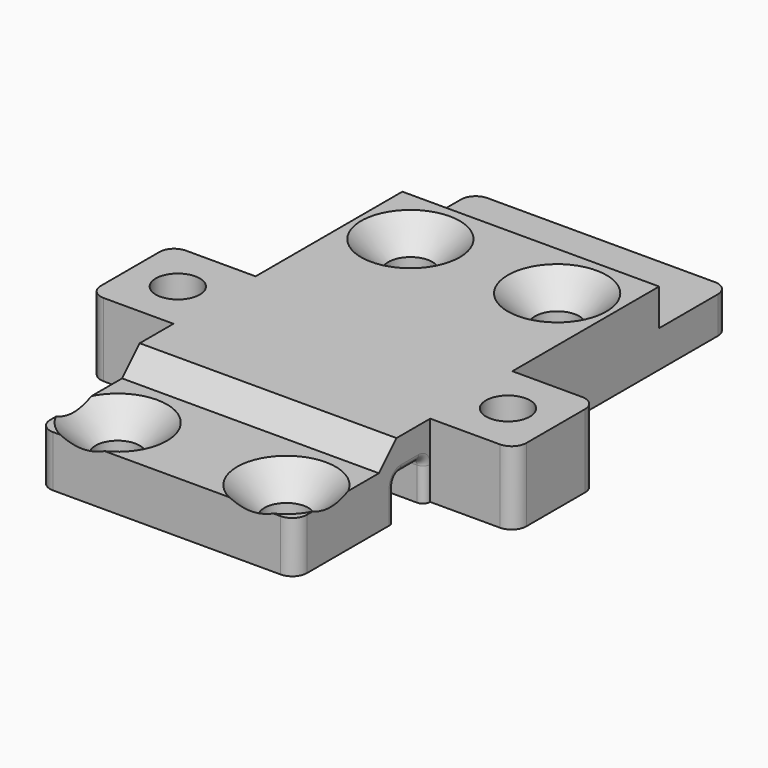
from build123d import *

# Parameters (mm, degrees)
F0_W            = 11.5
F0_H            = 14
F1_DEPTH        = 10
F2_W            = 5
F2_H            = 5.5
F2_H_2          = 4
F2_W_2          = 12
F2_H_3          = 5
F3_DEPTH        = 17.501
F7_D            = 5
F8_D            = 6
F9_D            = 6
F9_CSINK_D      = 13.44
F9_CSINK_ANGLE  = 90
F11_D           = 6
F11_CSINK_D     = 13.44
F11_CSINK_ANGLE = 90
F12_R           = 2
F13_R           = 0.99999


# Not quite as in the source:
# - a fillet or chamfer is up to 0.001 mm smaller than in the source, because OpenCascade refuses the exact size


with BuildPart() as f1:
    # F0 (on Top) → F1 (new body)
    with BuildSketch(Plane.XY):
        with Locations((23.25, 4.2037045646)):
            Rectangle(F0_W, F0_H)
        Polygon((17.5, 48.2037045646), (0, 48.2037045646), (0, -25.7962954354), (17.5, -25.7962954354), (17.5, -2.7962954354), (17.5, 11.2037045646), align=None)
    extrude(amount=F1_DEPTH)

    # F2 (on face) → F3 (cut, through all)
    with BuildSketch(Plane.YZ.offset(17.5)):
        Polygon((-25.7962954354, 10), (-25.7962954354, 7), (-11.5389361225, 7), (-8.5389361225, 10), align=None)
        with Locations((-6.2962954354, 2.75)):
            Rectangle(F2_W, F2_H)
        with Locations((13.7037045646, 2)):
            Rectangle(F2_W, F2_H_2)
        with Locations((42.2037045646, 7.5)):
            Rectangle(F2_W_2, F2_H_3)
    extrude(amount=-F3_DEPTH, mode=Mode.SUBTRACT)

    # F7 (through all)
    with Locations(Plane.XY.offset(5)):
        with Locations((10, 41.2037045646)):
            Hole(F7_D / 2)

    # F8 (through all)
    with Locations(Plane.XY.offset(10)):
        with Locations((22.5, 4.2037045646)):
            Hole(F8_D / 2)

    # F9 (through all)
    with Locations(Plane.XY.offset(7)):
        with Locations((11.5, -19.7962954354)):
            CounterSinkHole(F9_D / 2, F9_CSINK_D / 2, counter_sink_angle=F9_CSINK_ANGLE)

    # F11 (through all)
    with Locations(Plane.XY.offset(10)):
        with Locations((10, 28.2037045646)):
            CounterSinkHole(F11_D / 2, F11_CSINK_D / 2, counter_sink_angle=F11_CSINK_ANGLE)

    # F12
    f12_edges = [f1.edges().sort_by_distance(p)[0] for p in [
        (29, -2.796295, 5),
        (29, 11.203705, 5),
        (17.5, 48.203705, 2.5),
        (17.5, -25.796295, 3.5),
    ]]
    fillet(f12_edges, radius=F12_R)

    # F13 (radius 1 in the source; OpenCascade refuses exactly that, so slightly less here)
    f13_edges = [f1.edges().sort_by_distance(p)[0] for p in [
        (17.5, -6.296295, 5.5),
        (8.75, -3.796295, 5.5),
        (8.75, -8.796295, 5.5),
        (17.5, -8.796295, 2.75),
        (17.5, -3.796295, 2.75),
    ]]
    fillet(f13_edges, radius=F13_R)

    # F14: F1 across face


with BuildPart() as f1_1:
    add(f1.part)
    add(f1.part.mirror(Plane(origin=(0, 11.0999568472, 4.6658308471), x_dir=(0, -1, 0), z_dir=(-1, 0, 0))))


solid = f1_1.part
